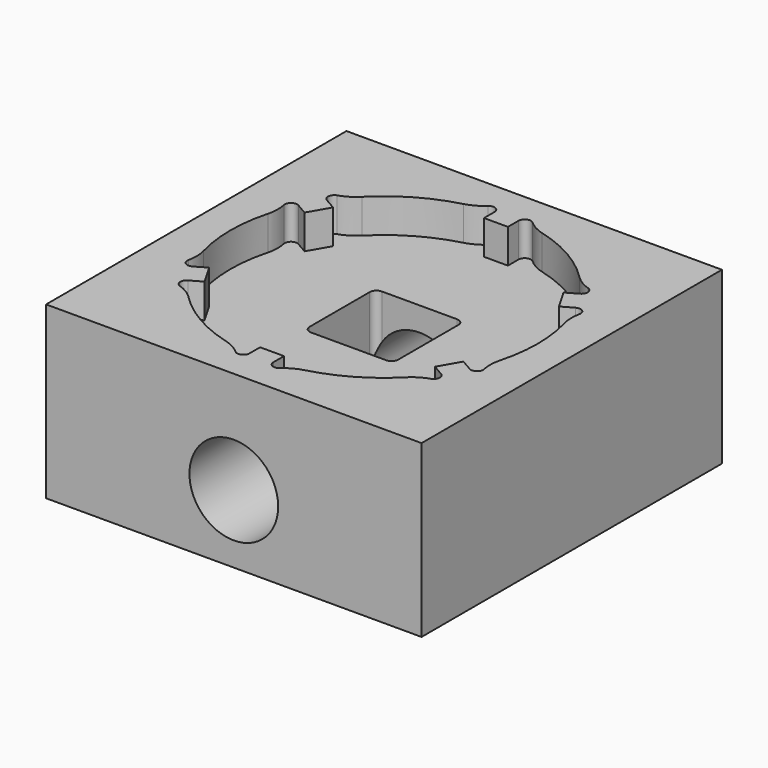
from build123d import *

# Parameters (mm, degrees)
F0_W     = 55
F0_H     = 55
F1_DEPTH = 25
F0_W_2   = 13
F0_H_2   = 13
F2_DEPTH = 20
F3_R     = 6
F4_R     = 1
F5_R     = 6.5
F6_DEPTH = 55.0010001


# Not quite as in the source:
# - a feature names something its author has since deleted; it is built from what else it names


with BuildPart() as f1:
    # F0 (on Top) → F1 (new body)
    with BuildSketch(Plane.XY):
        Rectangle(F0_W, F0_H)
        with BuildLine():
            ThreePointArc((-17.4666494059, 14.1833056278), (-11.25, 19.4855715851), (-3.5497782803, 22.2182149184))
            ThreePointArc((-3.5497782803, 22.2182149184), (-2.7701303651, 23.3380473177), (-1.75, 22.4318412084))
            Line((-1.75, 22.4318412084), (-1.75, 20.5))
            Line((-1.75, 20.5), (1.75, 20.5))
            Line((1.75, 20.5), (1.75, 22.4318412084))
            ThreePointArc((1.75, 22.4318412084), (2.7701303651, 23.3380473177), (3.5497782803, 22.2182149184))
            ThreePointArc((3.5497782803, 22.2182149184), (11.25, 19.4855715851), (17.4666494059, 14.1833056278))
            ThreePointArc((17.4666494059, 14.1833056278), (18.8262766693, 14.0680269268), (18.5515443402, 12.7314650608))
            Line((18.5515443402, 12.7314650608), (16.8785207776, 11.7655444566))
            Line((16.8785207776, 11.7655444566), (18.6285207776, 8.7344555434))
            Line((18.6285207776, 8.7344555434), (20.3015443402, 9.7003761476))
            ThreePointArc((20.3015443402, 9.7003761476), (21.5964070344, 9.2700203909), (21.0164276863, 8.0349092906))
            ThreePointArc((21.0164276863, 8.0349092906), (22.5, 0), (21.0164276863, -8.0349092906))
            ThreePointArc((21.0164276863, -8.0349092906), (21.5964070344, -9.2700203909), (20.3015443402, -9.7003761476))
            Line((20.3015443402, -9.7003761476), (18.6285207776, -8.7344555434))
            Line((18.6285207776, -8.7344555434), (16.8785207776, -11.7655444566))
            Line((16.8785207776, -11.7655444566), (18.5515443402, -12.7314650608))
            ThreePointArc((18.5515443402, -12.7314650608), (18.8262766693, -14.0680269268), (17.4666494059, -14.1833056278))
            ThreePointArc((17.4666494059, -14.1833056278), (11.25, -19.4855715851), (3.5497782803, -22.2182149184))
            ThreePointArc((3.5497782803, -22.2182149184), (2.7701303651, -23.3380473177), (1.75, -22.4318412084))
            Line((1.75, -22.4318412084), (1.75, -20.5))
            Line((1.75, -20.5), (-1.75, -20.5))
            Line((-1.75, -20.5), (-1.75, -22.4318412084))
            ThreePointArc((-1.75, -22.4318412084), (-2.7701303651, -23.3380473177), (-3.5497782803, -22.2182149184))
            ThreePointArc((-3.5497782803, -22.2182149184), (-11.25, -19.4855715851), (-17.4666494059, -14.1833056278))
            ThreePointArc((-17.4666494059, -14.1833056278), (-18.8262766693, -14.0680269268), (-18.5515443402, -12.7314650608))
            Line((-18.5515443402, -12.7314650608), (-16.8785207776, -11.7655444566))
            Line((-16.8785207776, -11.7655444566), (-18.6285207776, -8.7344555434))
            Line((-18.6285207776, -8.7344555434), (-20.3015443402, -9.7003761476))
            ThreePointArc((-20.3015443402, -9.7003761476), (-21.5964070344, -9.2700203909), (-21.0164276863, -8.0349092906))
            ThreePointArc((-21.0164276863, -8.0349092906), (-22.5, 0), (-21.0164276863, 8.0349092906))
            ThreePointArc((-21.0164276863, 8.0349092906), (-21.5964070344, 9.2700203909), (-20.3015443402, 9.7003761476))
            Line((-20.3015443402, 9.7003761476), (-18.6285207776, 8.7344555434))
            Line((-18.6285207776, 8.7344555434), (-16.8785207776, 11.7655444566))
            Line((-16.8785207776, 11.7655444566), (-18.5515443402, 12.7314650608))
            ThreePointArc((-18.5515443402, 12.7314650608), (-18.8262766693, 14.0680269268), (-17.4666494059, 14.1833056278))
        make_face(mode=Mode.SUBTRACT)
    extrude(amount=F1_DEPTH)

    # F0 (on Top) → F2 (join)
    with BuildSketch(Plane.XY):
        with BuildLine():
            ThreePointArc((-1.75, 22.4318412084), (-2.7701303651, 23.3380473177), (-3.5497782803, 22.2182149184))
            ThreePointArc((-3.5497782803, 22.2182149184), (-11.25, 19.4855715851), (-17.4666494059, 14.1833056278))
            ThreePointArc((-17.4666494059, 14.1833056278), (-18.8262766693, 14.0680269268), (-18.5515443402, 12.7314650608))
            Line((-18.5515443402, 12.7314650608), (-16.8785207776, 11.7655444566))
            Line((-16.8785207776, 11.7655444566), (-18.6285207776, 8.7344555434))
            Line((-18.6285207776, 8.7344555434), (-20.3015443402, 9.7003761476))
            ThreePointArc((-20.3015443402, 9.7003761476), (-21.5964070344, 9.2700203909), (-21.0164276863, 8.0349092906))
            ThreePointArc((-21.0164276863, 8.0349092906), (-22.5, 0), (-21.0164276863, -8.0349092906))
            ThreePointArc((-21.0164276863, -8.0349092906), (-21.5964070344, -9.2700203909), (-20.3015443402, -9.7003761476))
            Line((-20.3015443402, -9.7003761476), (-18.6285207776, -8.7344555434))
            Line((-18.6285207776, -8.7344555434), (-16.8785207776, -11.7655444566))
            Line((-16.8785207776, -11.7655444566), (-18.5515443402, -12.7314650608))
            ThreePointArc((-18.5515443402, -12.7314650608), (-18.8262766693, -14.0680269268), (-17.4666494059, -14.1833056278))
            ThreePointArc((-17.4666494059, -14.1833056278), (-11.25, -19.4855715851), (-3.5497782803, -22.2182149184))
            ThreePointArc((-3.5497782803, -22.2182149184), (-2.7701303651, -23.3380473177), (-1.75, -22.4318412084))
            Line((-1.75, -22.4318412084), (-1.75, -20.5))
            Line((-1.75, -20.5), (1.75, -20.5))
            Line((1.75, -20.5), (1.75, -22.4318412084))
            ThreePointArc((1.75, -22.4318412084), (2.7701303651, -23.3380473177), (3.5497782803, -22.2182149184))
            ThreePointArc((3.5497782803, -22.2182149184), (11.25, -19.4855715851), (17.4666494059, -14.1833056278))
            ThreePointArc((17.4666494059, -14.1833056278), (18.8262766693, -14.0680269268), (18.5515443402, -12.7314650608))
            Line((18.5515443402, -12.7314650608), (16.8785207776, -11.7655444566))
            Line((16.8785207776, -11.7655444566), (18.6285207776, -8.7344555434))
            Line((18.6285207776, -8.7344555434), (20.3015443402, -9.7003761476))
            ThreePointArc((20.3015443402, -9.7003761476), (21.5964070344, -9.2700203909), (21.0164276863, -8.0349092906))
            ThreePointArc((21.0164276863, -8.0349092906), (22.5, 0), (21.0164276863, 8.0349092906))
            ThreePointArc((21.0164276863, 8.0349092906), (21.5964070344, 9.2700203909), (20.3015443402, 9.7003761476))
            Line((20.3015443402, 9.7003761476), (18.6285207776, 8.7344555434))
            Line((18.6285207776, 8.7344555434), (16.8785207776, 11.7655444566))
            Line((16.8785207776, 11.7655444566), (18.5515443402, 12.7314650608))
            ThreePointArc((18.5515443402, 12.7314650608), (18.8262766693, 14.0680269268), (17.4666494059, 14.1833056278))
            ThreePointArc((17.4666494059, 14.1833056278), (11.25, 19.4855715851), (3.5497782803, 22.2182149184))
            ThreePointArc((3.5497782803, 22.2182149184), (2.7701303651, 23.3380473177), (1.75, 22.4318412084))
            Line((1.75, 22.4318412084), (1.75, 20.5))
            Line((1.75, 20.5), (-1.75, 20.5))
            Line((-1.75, 20.5), (-1.75, 22.4318412084))
        make_face()
        Rectangle(F0_W_2, F0_H_2, mode=Mode.SUBTRACT)
    extrude(amount=F2_DEPTH)

    # F3
    f3_edges = [f1.edges().sort_by_distance(p)[0] for p in [
        (-21.016428, -8.034909, 22.5),
        (-21.016428, 8.034909, 22.5),
        (-17.466649, 14.183306, 22.5),
        (-3.549778, 22.218215, 22.5),
        (-17.466649, -14.183306, 22.5),
        (-3.549778, -22.218215, 22.5),
        (17.466649, 14.183306, 22.5),
        (21.016428, 8.034909, 22.5),
        (21.016428, -8.034909, 22.5),
        (17.466649, -14.183306, 22.5),
        (3.549778, -22.218215, 22.5),
        (3.549778, 22.218215, 22.5),
    ]]
    fillet(f3_edges, radius=F3_R)

    # F4
    f4_edges = [f1.edges().sort_by_distance(p)[0] for p in [
        (6.5, 6.5, 10),
        (-6.5, 6.5, 10),
        (-6.5, -6.5, 10),
        (6.5, -6.5, 10),
    ]]
    fillet(f4_edges, radius=F4_R)

    # F5 (on face) → F6 (cut, through all)
    with BuildSketch(Plane.XZ.offset(27.5)):
        with Locations((0, 10)):
            Circle(F5_R)
    extrude(amount=-F6_DEPTH, mode=Mode.SUBTRACT)


solid = f1.part
